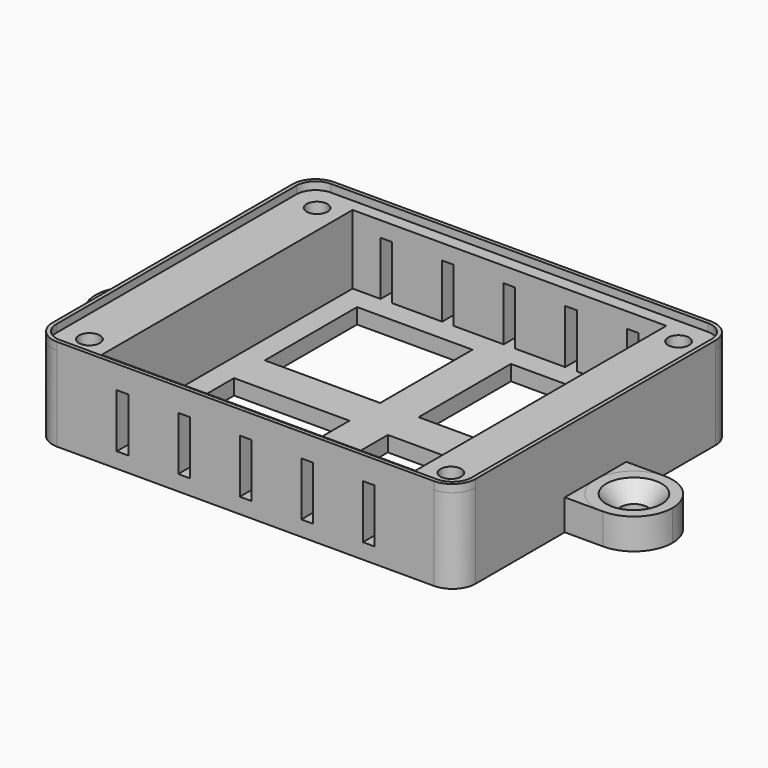
from build123d import *

# Parameters (mm, degrees)
F0_W              = 51.8
F0_H              = 51.8
F1_DEPTH          = 13.97
F2_DEPTH          = 5.08
F0_W_2            = 19.05
F0_H_2            = 19.05
F3_DEPTH          = 2.54
F4_R              = 3.81
F7_D              = 3.4544
F9_W              = 1.905
F9_H              = 8.89
F10_DEPTH         = 57.15
F11_DEPTH         = 5.08
F14_D             = 4.4958
F14_CSINK_D       = 9.1186
F14_CSINK_ANGLE   = 82
F14_2_D           = 4.4958
F14_2_CSINK_D     = 9.1186
F14_2_CSINK_ANGLE = 82
F16_DEPTH         = 1.27


# Not quite as in the source:
# - a feature names something its author has since deleted; it is built from what else it names


with BuildPart() as f1:
    # F0 (on Top) → F1 (new body)
    with BuildSketch(Plane.XY):
        Polygon((-34.925, -28.575), (34.925, -28.575), (34.925, -6.35), (34.925, 4.95e-08), (34.925, 6.35), (34.925, 28.575), (-34.925, 28.575), (-34.925, 6.35), (-34.925, 0), (-34.925, -6.35), align=None)
        Rectangle(F0_W, F0_H, mode=Mode.SUBTRACT)
    extrude(amount=F1_DEPTH)

    # F0 (on Top) → F2 (join)
    with BuildSketch(Plane.XY):
        with BuildLine():
            ThreePointArc((-41.275, 6.35), (-36.7848719395, 4.4901280605), (-34.925, 0))
            Line((-34.925, 0), (-34.925, 6.35))
            Line((-34.925, 6.35), (-41.275, 6.35))
        make_face()
        with BuildLine():
            Line((34.925, 6.35), (34.925, 4.95e-08))
            ThreePointArc((34.925, 4.95e-08), (36.784871957, 4.490128078), (41.275, 6.35))
            Line((41.275, 6.35), (34.925, 6.35))
        make_face()
        with BuildLine():
            Line((34.925, 4.95e-08), (34.925, -6.35))
            Line((34.925, -6.35), (41.275, -6.35))
            ThreePointArc((41.275, -6.35), (36.784871922, -4.490128043), (34.925, 4.95e-08))
        make_face()
        with BuildLine():
            Line((-41.275, -6.35), (-34.925, -6.35))
            Line((-34.925, -6.35), (-34.925, 0))
            ThreePointArc((-34.925, 0), (-36.7848719395, -4.4901280605), (-41.275, -6.35))
        make_face()
    extrude(amount=F2_DEPTH)

    # F0 (on Top) → F3 (join)
    with BuildSketch(Plane.XY):
        Rectangle(F0_W, F0_H)
        with Locations((-12.7, -12.7)):
            Rectangle(F0_W_2, F0_H_2, mode=Mode.SUBTRACT)
        with Locations((12.7, -12.7)):
            Rectangle(F0_W_2, F0_H_2, mode=Mode.SUBTRACT)
        with Locations((-12.7, 12.7)):
            Rectangle(F0_W_2, F0_H_2, mode=Mode.SUBTRACT)
        with Locations((12.7, 12.7)):
            Rectangle(F0_W_2, F0_H_2, mode=Mode.SUBTRACT)
    extrude(amount=F3_DEPTH)

    # F4
    f4_edges = [f1.edges().sort_by_distance(p)[0] for p in [
        (-34.925, -28.575, 6.985),
        (34.925, 28.575, 6.985),
        (34.925, -28.575, 6.985),
        (-34.925, 28.575, 6.985),
    ]]
    fillet(f4_edges, radius=F4_R)

    # F7 (through all)
    with Locations(Plane.XY.offset(13.97)):
        with Locations((-29.845, 23.495), (-29.845, -23.495), (29.845, -23.495), (29.845, 23.495)):
            Hole(F7_D / 2)

    # F9 (on offset) → F10 (cut)
    with BuildSketch(Plane.XZ.offset(28.575)):
        with Locations((10.16, 6.985)):
            Rectangle(F9_W, F9_H)
        with Locations((0, 6.985)):
            Rectangle(F9_W, F9_H)
        with Locations((-20.3200003028, 6.985)):
            Rectangle(F9_W, F9_H)
        with Locations((-10.1600001514, 6.985)):
            Rectangle(F9_W, F9_H)
        with Locations((20.32, 6.985)):
            Rectangle(F9_W, F9_H)
    extrude(amount=-F10_DEPTH, mode=Mode.SUBTRACT)

    # F15 (on face) → F16 (join)
    with BuildSketch(Plane.XY.offset(13.97)):
        with BuildLine():
            ThreePointArc((-34.925, -24.765), (-33.8090768363, -27.4590768363), (-31.115, -28.575))
            Line((-31.115, -28.575), (31.115, -28.575))
            ThreePointArc((31.115, -28.575), (33.8090768363, -27.4590768363), (34.925, -24.765))
            Line((34.925, -24.765), (34.925, 24.765))
            ThreePointArc((34.925, 24.765), (33.8090768363, 27.4590768363), (31.115, 28.575))
            Line((31.115, 28.575), (-31.115, 28.575))
            ThreePointArc((-31.115, 28.575), (-33.8090768363, 27.4590768363), (-34.925, 24.765))
            Line((-34.925, 24.765), (-34.925, -24.765))
        make_face()
        with BuildLine():
            Line((34.29, 24.765), (34.29, -24.765))
            ThreePointArc((34.29, -24.765), (33.3600640303, -27.0100640303), (31.115, -27.94))
            Line((31.115, -27.94), (-31.115, -27.94))
            ThreePointArc((-31.115, -27.94), (-33.3600640303, -27.0100640303), (-34.29, -24.765))
            Line((-34.29, -24.765), (-34.29, 24.765))
            ThreePointArc((-34.29, 24.765), (-33.3600640303, 27.0100640303), (-31.115, 27.94))
            Line((-31.115, 27.94), (31.115, 27.94))
            ThreePointArc((31.115, 27.94), (33.3600640303, 27.0100640303), (34.29, 24.765))
        make_face(mode=Mode.SUBTRACT)
    extrude(amount=F16_DEPTH)


with BuildPart() as f11:
    # F0 (on Top) → F11 (new body)
    with BuildSketch(Plane.XY):
        with BuildLine():
            ThreePointArc((41.275, 6.35), (36.784871957, 4.490128078), (34.925, 4.95e-08))
            ThreePointArc((34.925, 4.95e-08), (36.784871922, -4.490128043), (41.275, -6.35))
            ThreePointArc((41.275, -6.35), (45.7651280605, -4.4901280605), (47.625, 0))
            ThreePointArc((47.625, 0), (45.7651280605, 4.4901280605), (41.275, 6.35))
        make_face()
    extrude(amount=F11_DEPTH)

    # F14 (through all)
    with Locations(Plane.XY.offset(5.08)):
        with Locations((-41.275, 0), (41.275, 0)):
            CounterSinkHole(F14_D / 2, F14_CSINK_D / 2, counter_sink_angle=F14_CSINK_ANGLE)


with BuildPart() as f11b:
    # F0 (on Top) → F11, piece 2 (new body)
    with BuildSketch(Plane.XY):
        with BuildLine():
            ThreePointArc((-41.275, -6.35), (-36.7848719395, -4.4901280605), (-34.925, 0))
            ThreePointArc((-34.925, 0), (-36.7848719395, 4.4901280605), (-41.275, 6.35))
            ThreePointArc((-41.275, 6.35), (-47.625, 0), (-41.275, -6.35))
        make_face()
    extrude(amount=F11_DEPTH)

    # F14#2 (through all)
    with Locations(Plane.XY.offset(5.08)):
        with Locations((-41.275, 0), (41.275, 0)):
            CounterSinkHole(F14_2_D / 2, F14_2_CSINK_D / 2, counter_sink_angle=F14_2_CSINK_ANGLE)


solid = Compound([f1.part, f11.part, f11b.part])
